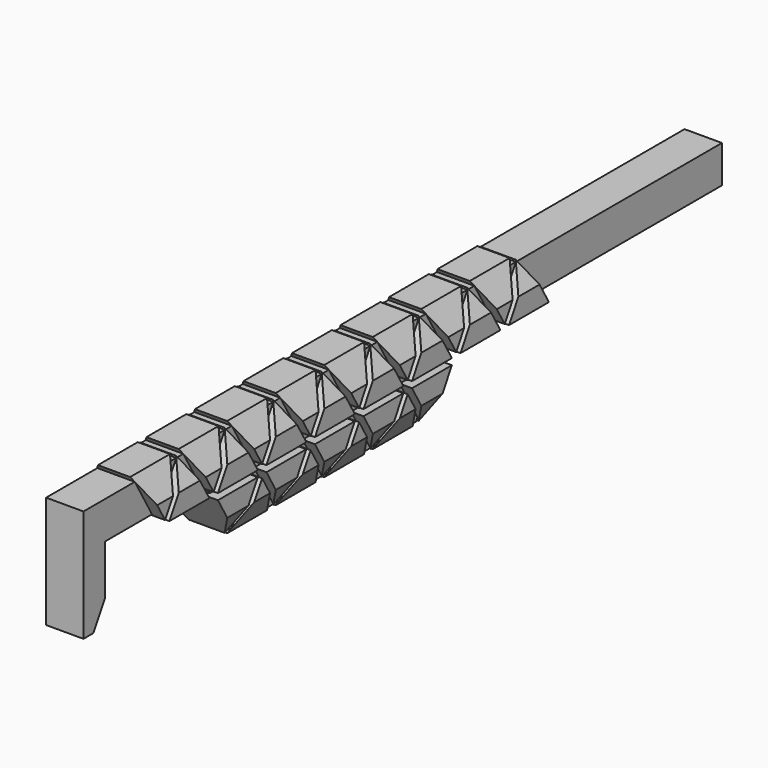
from build123d import *

# Parameters (mm, degrees)
F1_W     = 3.175
F1_H     = 9.525
F2_DEPTH = 9.525
F1_W_2   = 179.4027834434
F1_H_2   = 19.05
F3_DEPTH = 9.525
F4_DEPTH = 15.875
F6_DEPTH = 177.8


with BuildPart() as f2:
    # F1 (on Right) → F2 (new body, symmetric)
    with BuildSketch(Plane.YZ):
        Polygon((-37.7075152621, 2.2672726281), (-48.7060378902, 21.3172726281), (-139.5049298612, 21.3172726281), (-139.5049298612, -35.8327273719), (-133.1549298612, -35.8327273719), (-125.8225814425, -23.1327273719), (-125.8225814425, 2.2672726281), (-62.3225814425, 2.2672726281), align=None)
        Polygon((-29.5902419379, 2.2672726281), (-18.5917193098, 21.3172726281), (-48.7060378902, 21.3172726281), (-37.7075152621, 2.2672726281), align=None)
        Polygon((-6.8082628621, 2.2672726281), (-17.8067854902, 21.3172726281), (-18.5917193098, 21.3172726281), (-29.5902419379, 2.2672726281), align=None)
        Polygon((9.950378257, 17.2345606957), (9.950378257, 21.3172726281), (-17.8067854902, 21.3172726281), (-6.8082628621, 2.2672726281), (1.3090104621, 2.2672726281), align=None)
        Polygon((13.125378257, 21.2602685025), (13.125378257, 11.7922726281), (13.125378257, 2.2672726281), (24.0909895379, 2.2672726281), align=None)
        with Locations((11.537878257, 7.0297726281)):
            Rectangle(F1_W, F1_H)
        Polygon((12.3075330902, 21.3172726281), (9.950378257, 17.2345606957), (9.950378257, 11.7922726281), (13.125378257, 11.7922726281), (13.125378257, 21.2602685025), (13.0924669098, 21.3172726281), align=None)
        Polygon((9.950378257, 11.7922726281), (9.950378257, 17.2345606957), (1.3090104621, 2.2672726281), (9.950378257, 2.2672726281), align=None)
        Polygon((12.3075330902, 21.3172726281), (9.950378257, 21.3172726281), (9.950378257, 17.2345606957), align=None)
        Polygon((13.125378257, 21.3172726281), (13.125378257, 21.2602685025), (24.0909895379, 2.2672726281), (87.7225948136, 2.2672726281), (87.7225948136, 21.3172726281), align=None)
        Polygon((0, 0), (1.3090104621, 2.2672726281), (-6.8082628621, 2.2672726281), (-5.4992524, 0), (-30.8992524, 0), (-29.5902419379, 2.2672726281), (-37.7075152621, 2.2672726281), (-62.3225814425, 2.2672726281), (-51.9763694491, -15.6528922105), (-47.7894943379, -22.9047726281), (-42.7485048, -14.1735226281), (-41.3736894715, -14.9672726281), (-44.8405059529, -24.4922726281), (-34.4873710954, -24.4922726281), (47.6579024332, -24.4922726281), (72.2729641566, -24.4922726281), (87.7225948136, 2.2672726281), (24.0909895379, 2.2672726281), (25.4, 0), (9.950378257, 0), align=None)
        Polygon((13.125378257, 2.2672726281), (9.950378257, 2.2672726281), (9.950378257, 0), (25.4, 0), (24.0909895379, 2.2672726281), align=None)
        Polygon((9.950378257, 2.2672726281), (1.3090104621, 2.2672726281), (0, 0), (9.950378257, 0), align=None)
        Polygon((-5.4992524, 0), (-6.8082628621, 2.2672726281), (-29.5902419379, 2.2672726281), (-30.8992524, 0), align=None)
        Polygon((-42.7485048, -14.1735226281), (-47.7894943379, -22.9047726281), (-46.8729507855, -24.4922726281), (-44.8405059529, -24.4922726281), (-41.3736894715, -14.9672726281), align=None)
    extrude(amount=F2_DEPTH, both=True)


with BuildPart() as f3:
    # F1 (on Right) → F3 (new body, symmetric)
    with BuildSketch(Plane.YZ):
        with Locations((177.4239865353, 11.7922726281)):
            Rectangle(F1_W_2, F1_H_2)
    extrude(amount=F3_DEPTH, both=True)


with BuildPart() as f4:
    # F0 (on Right) → F4 (new body, symmetric)
    with BuildSketch(Plane.YZ):
        Polygon((102.648144371, 23.5845452561), (77.248144371, 23.5845452561), (89.948144371, 1.5875), align=None)
    extrude(amount=F4_DEPTH, both=True)


with BuildPart() as f4b:
    # F0 (on Right) → F4, piece 2 (new body, symmetric)
    with BuildSketch(Plane.YZ):
        Polygon((61.798513714, 0), (87.198513714, 0), (74.498513714, 21.9970452561), align=None)
    extrude(amount=F4_DEPTH, both=True)


with BuildPart() as f4c:
    # F0 (on Right) → F4, piece 3 (new body, symmetric)
    with BuildSketch(Plane.YZ):
        Polygon((74.498513714, -25.1720452561), (87.198513714, -3.175), (61.798513714, -3.175), align=None)
    extrude(amount=F4_DEPTH, both=True)


with BuildPart() as f4d:
    # F0 (on Right) → F4, piece 4 (new body, symmetric)
    with BuildSketch(Plane.YZ):
        Polygon((71.748891971, -26.7595452561), (59.048891971, -4.7625), (46.348891971, -26.7595452561), align=None)
    extrude(amount=F4_DEPTH, both=True)


with BuildPart() as f4e:
    # F0 (on Right) → F4, piece 5 (new body, symmetric)
    with BuildSketch(Plane.YZ):
        Polygon((56.299261314, -3.175), (30.899261314, -3.175), (43.599261314, -25.1720452561), align=None)
    extrude(amount=F4_DEPTH, both=True)


with BuildPart() as f4f:
    # F0 (on Right) → F4, piece 6 (new body, symmetric)
    with BuildSketch(Plane.YZ):
        Polygon((46.348891971, 23.5845452561), (59.048891971, 1.5875), (71.748891971, 23.5845452561), align=None)
    extrude(amount=F4_DEPTH, both=True)


with BuildPart() as f4g:
    # F0 (on Right) → F4, piece 7 (new body, symmetric)
    with BuildSketch(Plane.YZ):
        Polygon((43.599261314, 21.9970452561), (30.899261314, 0), (43.599261314, 0), (56.299261314, 0), align=None)
    extrude(amount=F4_DEPTH, both=True)


with BuildPart() as f4h:
    # F0 (on Right) → F4, piece 8 (new body, symmetric)
    with BuildSketch(Plane.YZ):
        Polygon((40.849630657, -26.7595452561), (28.149630657, -4.7625), (15.449630657, -26.7595452561), align=None)
    extrude(amount=F4_DEPTH, both=True)


with BuildPart() as f4i:
    # F0 (on Right) → F4, piece 9 (new body, symmetric)
    with BuildSketch(Plane.YZ):
        Polygon((15.449630657, 23.5845452561), (28.149630657, 1.5875), (40.849630657, 23.5845452561), align=None)
    extrude(amount=F4_DEPTH, both=True)


with BuildPart() as f4j:
    # F0 (on Right) → F4, piece 10 (new body, symmetric)
    with BuildSketch(Plane.YZ):
        Polygon((12.7, 21.9970452561), (0, 0), (25.4, 0), align=None)
    extrude(amount=F4_DEPTH, both=True)


with BuildPart() as f4k:
    # F0 (on Right) → F4, piece 11 (new body, symmetric)
    with BuildSketch(Plane.YZ):
        Polygon((25.4, -3.175), (0, -3.175), (12.7, -25.1720452561), align=None)
    extrude(amount=F4_DEPTH, both=True)


with BuildPart() as f4l:
    # F0 (on Right) → F4, piece 12 (new body, symmetric)
    with BuildSketch(Plane.YZ):
        Polygon((9.950378257, -26.7595452561), (-2.749621743, -4.7625), (-15.449621743, -26.7595452561), align=None)
    extrude(amount=F4_DEPTH, both=True)


with BuildPart() as f4m:
    # F0 (on Right) → F4, piece 13 (new body, symmetric)
    with BuildSketch(Plane.YZ):
        Polygon((-15.449621743, 23.5845452561), (-2.749621743, 1.5875), (9.950378257, 23.5845452561), align=None)
    extrude(amount=F4_DEPTH, both=True)


with BuildPart() as f4n:
    # F0 (on Right) → F4, piece 14 (new body, symmetric)
    with BuildSketch(Plane.YZ):
        Polygon((-18.1992524, 21.9970452561), (-30.8992524, 0), (-5.4992524, 0), align=None)
    extrude(amount=F4_DEPTH, both=True)


with BuildPart() as f4o:
    # F0 (on Right) → F4, piece 15 (new body, symmetric)
    with BuildSketch(Plane.YZ):
        Polygon((-5.4992524, -3.175), (-30.8992524, -3.175), (-18.1992524, -25.1720452561), align=None)
    extrude(amount=F4_DEPTH, both=True)


with BuildPart() as f4p:
    # F0 (on Right) → F4, piece 16 (new body, symmetric)
    with BuildSketch(Plane.YZ):
        Polygon((-20.948874143, -26.7595452561), (-33.648874143, -4.7625), (-46.348874143, -26.7595452561), align=None)
    extrude(amount=F4_DEPTH, both=True)


with BuildPart() as f4q:
    # F0 (on Right) → F4, piece 17 (new body, symmetric)
    with BuildSketch(Plane.YZ):
        Polygon((-46.348874143, 23.5845452561), (-33.648874143, 1.5875), (-20.948874143, 23.5845452561), align=None)
    extrude(amount=F4_DEPTH, both=True)


with BuildPart() as f4r:
    # F0 (on Right) → F4, piece 18 (new body, symmetric)
    with BuildSketch(Plane.YZ):
        Polygon((-49.0985048, 21.9970452561), (-61.7985048, 0), (-36.3985048, 0), align=None)
    extrude(amount=F4_DEPTH, both=True)


with BuildPart() as f4s:
    # F0 (on Right) → F4, piece 19 (new body, symmetric)
    with BuildSketch(Plane.YZ):
        Polygon((-36.3985048, -3.175), (-61.7985048, -3.175), (-49.0985048, -25.1720452561), align=None)
    extrude(amount=F4_DEPTH, both=True)


with BuildPart() as f4t:
    # F0 (on Right) → F4, piece 20 (new body, symmetric)
    with BuildSketch(Plane.YZ):
        Polygon((-77.248126543, 23.5845452561), (-64.548126543, 1.5875), (-51.848126543, 23.5845452561), align=None)
    extrude(amount=F4_DEPTH, both=True)


with BuildPart() as f4u:
    # F0 (on Right) → F4, piece 21 (new body, symmetric)
    with BuildSketch(Plane.YZ):
        Polygon((-92.6977572, 0), (-67.2977572, 0), (-79.9977572, 21.9970452561), align=None)
    extrude(amount=F4_DEPTH, both=True)


with BuildPart() as f4v:
    # F0 (on Right) → F4, piece 22 (new body, symmetric)
    with BuildSketch(Plane.YZ):
        Polygon((-95.447378943, 1.5875), (-82.747378943, 23.5845452561), (-108.147378943, 23.5845452561), align=None)
    extrude(amount=F4_DEPTH, both=True)


with BuildPart() as f4w:
    # F0 (on Right) → F4, piece 23 (new body, symmetric)
    with BuildSketch(Plane.YZ):
        Polygon((92.697766114, 0), (118.097766114, 0), (105.397766114, 21.9970452561), align=None)
    extrude(amount=F4_DEPTH, both=True)


with BuildPart() as f4x:
    # F0 (on Right) → F4, piece 24 (new body, symmetric)
    with BuildSketch(Plane.YZ):
        Polygon((133.547396771, 23.5845452561), (108.147396771, 23.5845452561), (120.847396771, 1.5875), align=None)
    extrude(amount=F4_DEPTH, both=True)


with BuildPart() as f4y:
    # F0 (on Right) → F4, piece 25 (new body, symmetric)
    with BuildSketch(Plane.YZ):
        Polygon((123.597018514, 0), (148.997018514, 0), (136.297018514, 21.9970452561), align=None)
    extrude(amount=F4_DEPTH, both=True)


with BuildPart() as f6_tool:
    # F5 (on Front) → F6 (new body, symmetric)
    with BuildSketch(Plane.XZ):
        Polygon((8.2159895379, -26.7595452561), (15.875, -26.7595452561), (15.875, -13.49375), (9.525, -24.4922726281), align=None)
        Polygon((-15.875, -26.7595452561), (-8.2159895379, -26.7595452561), (-9.525, -24.4922726281), (-15.875, -13.49375), align=None)
        Polygon((-9.525, 21.3172726281), (-8.2159895379, 23.5845452561), (-15.875, 23.5845452561), (-15.875, 10.31875), align=None)
        Polygon((15.875, 10.31875), (15.875, 23.5845452561), (8.2159895379, 23.5845452561), (9.525, 21.3172726281), align=None)
    extrude(amount=F6_DEPTH, both=True)


with BuildPart() as f4_1:
    add(f4.part)

    # F6: cut by f6_tool
    add(f6_tool.part, mode=Mode.SUBTRACT)


with BuildPart() as f4b_1:
    add(f4b.part)

    # F6: cut by f6_tool
    add(f6_tool.part, mode=Mode.SUBTRACT)


with BuildPart() as f4c_1:
    add(f4c.part)

    # F6: cut by f6_tool
    add(f6_tool.part, mode=Mode.SUBTRACT)


with BuildPart() as f4d_1:
    add(f4d.part)

    # F6: cut by f6_tool
    add(f6_tool.part, mode=Mode.SUBTRACT)


with BuildPart() as f4e_1:
    add(f4e.part)

    # F6: cut by f6_tool
    add(f6_tool.part, mode=Mode.SUBTRACT)


with BuildPart() as f4f_1:
    add(f4f.part)

    # F6: cut by f6_tool
    add(f6_tool.part, mode=Mode.SUBTRACT)


with BuildPart() as f4g_1:
    add(f4g.part)

    # F6: cut by f6_tool
    add(f6_tool.part, mode=Mode.SUBTRACT)


with BuildPart() as f4h_1:
    add(f4h.part)

    # F6: cut by f6_tool
    add(f6_tool.part, mode=Mode.SUBTRACT)


with BuildPart() as f4i_1:
    add(f4i.part)

    # F6: cut by f6_tool
    add(f6_tool.part, mode=Mode.SUBTRACT)


with BuildPart() as f4j_1:
    add(f4j.part)

    # F6: cut by f6_tool
    add(f6_tool.part, mode=Mode.SUBTRACT)


with BuildPart() as f4k_1:
    add(f4k.part)

    # F6: cut by f6_tool
    add(f6_tool.part, mode=Mode.SUBTRACT)


with BuildPart() as f4l_1:
    add(f4l.part)

    # F6: cut by f6_tool
    add(f6_tool.part, mode=Mode.SUBTRACT)


with BuildPart() as f4m_1:
    add(f4m.part)

    # F6: cut by f6_tool
    add(f6_tool.part, mode=Mode.SUBTRACT)


with BuildPart() as f4n_1:
    add(f4n.part)

    # F6: cut by f6_tool
    add(f6_tool.part, mode=Mode.SUBTRACT)


with BuildPart() as f4o_1:
    add(f4o.part)

    # F6: cut by f6_tool
    add(f6_tool.part, mode=Mode.SUBTRACT)


with BuildPart() as f4p_1:
    add(f4p.part)

    # F6: cut by f6_tool
    add(f6_tool.part, mode=Mode.SUBTRACT)


with BuildPart() as f4q_1:
    add(f4q.part)

    # F6: cut by f6_tool
    add(f6_tool.part, mode=Mode.SUBTRACT)


with BuildPart() as f4r_1:
    add(f4r.part)

    # F6: cut by f6_tool
    add(f6_tool.part, mode=Mode.SUBTRACT)


with BuildPart() as f4s_1:
    add(f4s.part)

    # F6: cut by f6_tool
    add(f6_tool.part, mode=Mode.SUBTRACT)


with BuildPart() as f4t_1:
    add(f4t.part)

    # F6: cut by f6_tool
    add(f6_tool.part, mode=Mode.SUBTRACT)


with BuildPart() as f4u_1:
    add(f4u.part)

    # F6: cut by f6_tool
    add(f6_tool.part, mode=Mode.SUBTRACT)


with BuildPart() as f4v_1:
    add(f4v.part)

    # F6: cut by f6_tool
    add(f6_tool.part, mode=Mode.SUBTRACT)


with BuildPart() as f4w_1:
    add(f4w.part)

    # F6: cut by f6_tool
    add(f6_tool.part, mode=Mode.SUBTRACT)


with BuildPart() as f4x_1:
    add(f4x.part)

    # F6: cut by f6_tool
    add(f6_tool.part, mode=Mode.SUBTRACT)


with BuildPart() as f4y_1:
    add(f4y.part)

    # F6: cut by f6_tool
    add(f6_tool.part, mode=Mode.SUBTRACT)


solid = Compound([f2.part, f3.part, f4_1.part, f4b_1.part, f4c_1.part, f4d_1.part, f4e_1.part, f4f_1.part, f4g_1.part, f4h_1.part, f4i_1.part, f4j_1.part, f4k_1.part, f4l_1.part, f4m_1.part, f4n_1.part, f4o_1.part, f4p_1.part, f4q_1.part, f4r_1.part, f4s_1.part, f4t_1.part, f4u_1.part, f4v_1.part, f4w_1.part, f4x_1.part, f4y_1.part])
